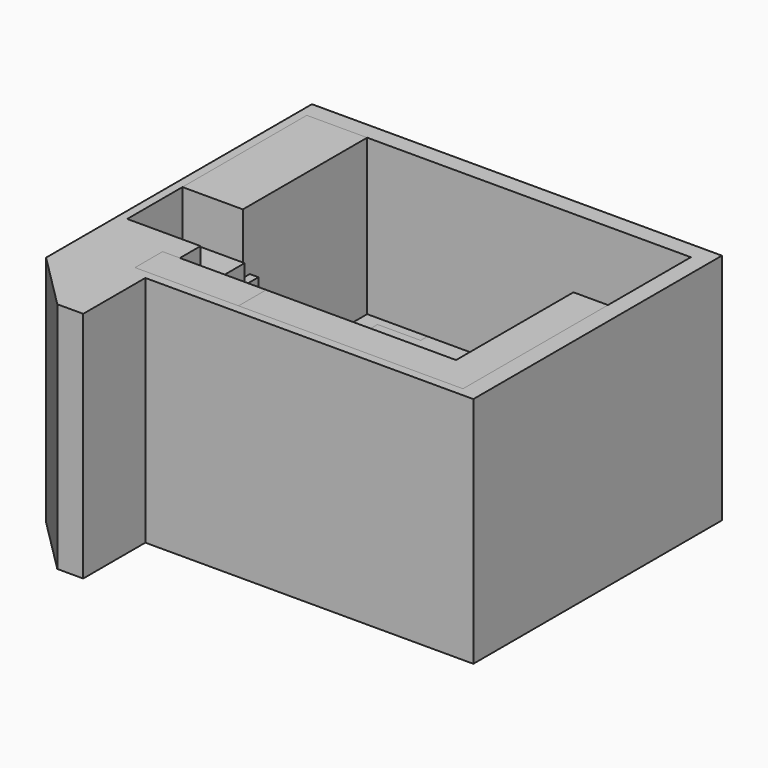
from build123d import *

# Parameters (mm, degrees)
F1_DEPTH       = 2700
F2_W           = 700
F2_H           = 2700
F3_DEPTH       = 1800
F4_W           = 500
F4_H           = 400
F5_DEPTH       = 750
F6_W           = 600
F6_H           = 900
F7_DEPTH       = 1200
F9_DEPTH       = 2100
F11_DEPTH      = 2000
F11_DEPTH_BACK = 200
F13_DEPTH      = 1200
F14_W          = 3850
F14_H          = 600
F15_DEPTH      = 900
F14_W_2        = 800
F14_H_2        = 900
F16_DEPTH      = 2000
F17_W          = 400
F17_H          = 400
F17_W_2        = 900
F17_W_3        = 500
F17_H_2        = 700
F17_H_3        = 100
F17_H_4        = 500
F18_DEPTH      = 2225
F17_H_5        = 300
F17_W_4        = 800
F17_H_6        = 1000
F17_W_5        = 450
F19_DEPTH      = 900
F17_W_6        = 300
F17_H_7        = 200


with BuildPart() as f1:
    # F0 (on Top) → F1 (new body)
    with BuildSketch(Plane.XY):
        Polygon((-1375, -2658.0309391022), (-1375, -1758.0309391022), (2425, -1758.0309391022), (2425, 1841.9690608978), (-2325, 1841.9690608978), (-2325, -2008.0309391022), (-1675, -2658.0309391022), align=None)
        Polygon((-2225, -958.0309391022), (-2225, 1641.9690608978), (2225, 1641.9690608978), (2225, -1658.0309391022), (-1375, -1658.0309391022), (-1375, -958.0309391022), align=None, mode=Mode.SUBTRACT)
    extrude(amount=F1_DEPTH)


with BuildPart() as f3:
    # F2 (on face) → F3 (new body)
    with BuildSketch(Plane.XZ.offset(-1641.9690608978)):
        with Locations((-1875, 1350)):
            Rectangle(F2_W, F2_H)
    extrude(amount=F3_DEPTH)


with BuildPart() as f5:
    # F4 (on Top) → F5 (new body)
    with BuildSketch(Plane.XY):
        with Locations((-325, -50)):
            Rectangle(F4_W, F4_H)
        Polygon((825, 300), (-75, 300), (-75, 150), (-75, -250), (-75, -400), (825, -400), (825, -250), (825, 150), align=None)
        with Locations((1075, -50)):
            Rectangle(F4_W, F4_H)
        Polygon((825, -400), (-75, -400), (-75, -550), (-75, -950), (-75, -1100), (825, -1100), (825, -950), (825, -550), align=None)
        with Locations((-325, -750)):
            Rectangle(F4_W, F4_H)
        with Locations((1075, -750)):
            Rectangle(F4_W, F4_H)
    extrude(amount=F5_DEPTH)


with BuildPart() as f7:
    # F6 (on face) → F7 (new body)
    with BuildSketch(Plane.XZ.offset(-1641.9690608978)):
        with Locations((1925, 450)):
            Rectangle(F6_W, F6_H)
    extrude(amount=F7_DEPTH)


with BuildPart() as f9:
    # F8 (on face) → F9 (new body, through all)
    with BuildSketch(Plane.XZ.offset(-441.9690608978)):
        Polygon((2215, 900), (2225, 900), (2225, 2700), (1825, 2700), (1825, 1500), (2215, 1500), align=None)
        Polygon((1625, 0), (2225, 0), (2225, 900), (2215, 900), (1625, 900), align=None)
    extrude(amount=F9_DEPTH)

    # F10 (on face) → F11 (join, two sides)
    with BuildSketch(Plane(origin=(1625, 0, 0), x_dir=(0, -1, 0), z_dir=(-1, 0, 0))) as f11_sk:
        Polygon((1648.0309391022, 900), (1658.0309391022, 900), (1658.0309391022, 2700), (1258.0309391022, 2700), (1258.0309391022, 1500), (1648.0309391022, 1500), align=None)
        Polygon((1258.0309391022, 0), (1658.0309391022, 0), (1658.0309391022, 900), (1648.0309391022, 900), (1258.0309391022, 900), align=None)
    extrude(amount=F11_DEPTH)
    extrude(f11_sk.sketch, amount=-F11_DEPTH_BACK)


with BuildPart() as f13:
    # F12 (on face) → F13 (new body)
    with BuildSketch(Plane(origin=(-375, 0, 0), x_dir=(0, -1, 0), z_dir=(-1, 0, 0))):
        Polygon((1658.0309391022, 0), (1658.0309391022, 2700), (1258.0309391022, 2700), (1258.0309391022, 1500), (1648.0309391022, 1500), (1648.0309391022, 900), (1258.0309391022, 900), (1258.0309391022, 0), align=None)
    extrude(amount=F13_DEPTH)


with BuildPart() as f15:
    # F14 (on Top) → F15 (new body)
    with BuildSketch(Plane.XY):
        with Locations((-300, 1341.9690608978)):
            Rectangle(F14_W, F14_H)
    extrude(amount=F15_DEPTH)


with BuildPart() as f16:
    # F14 (on Top) → F16 (new body)
    with BuildSketch(Plane.XY):
        with Locations((-1825, -508.0309391022)):
            Rectangle(F14_W_2, F14_H_2)
    extrude(amount=F16_DEPTH)


with BuildPart() as f18:
    # F17 (on Top) → F18 (new body)
    with BuildSketch(Plane.XY):
        with Locations((-75, -1458.0309391022)):
            Rectangle(F17_W, F17_H)
        with Locations((575, -1458.0309391022)):
            Rectangle(F17_W_2, F17_H)
        with Locations((1275, -1458.0309391022)):
            Rectangle(F17_W_3, F17_H)
        Polygon((1725, -1058.0309391022), (1525, -1258.0309391022), (1525, -1658.0309391022), (2225, -1658.0309391022), (2225, -1058.0309391022), align=None)
        Polygon((1825, -958.0309391022), (1725, -1058.0309391022), (2225, -1058.0309391022), (2225, -958.0309391022), align=None)
        with Locations((2025, -608.0309391022)):
            Rectangle(F17_W, F17_H_2)
        with Locations((2025, -208.0309391022)):
            Rectangle(F17_W, F17_H_3)
        with Locations((2025, 91.9690608978)):
            Rectangle(F17_W, F17_H_4)
    extrude(amount=F18_DEPTH)


with BuildPart() as f18b:
    # F17 (on Top) → F18, piece 2 (new body)
    with BuildSketch(Plane.XY):
        with Locations((2025, 791.9690608978)):
            Rectangle(F17_W, F17_H_5)
    extrude(amount=F18_DEPTH)


with BuildPart() as f18c:
    # F17 (on Top) → F18, piece 3 (new body)
    with BuildSketch(Plane.XY):
        with Locations((2025, 1391.9690608978)):
            Rectangle(F17_W, F17_H_3)
    extrude(amount=F18_DEPTH)


with BuildPart() as f18d:
    # F17 (on Top) → F18, piece 4 (new body)
    with BuildSketch(Plane.XY):
        with Locations((-1825, -608.0309391022)):
            Rectangle(F17_W_4, F17_H_2)
    extrude(amount=F18_DEPTH)


with BuildPart() as f18e:
    # F17 (on Top) → F18, piece 5 (new body)
    with BuildSketch(Plane.XY):
        with Locations((-2025, 1141.9690608978)):
            Rectangle(F17_W, F17_H_6)
    extrude(amount=F18_DEPTH)


with BuildPart() as f19:
    # F17 (on Top) → F19 (new body)
    with BuildSketch(Plane.XY):
        with Locations((-1075, 1291.9690608978)):
            Rectangle(F17_W_3, F17_H_4)
        with Locations((-600, 1591.9690608978)):
            Rectangle(F17_W_5, F17_H_3)
        with Locations((-150, 1591.9690608978)):
            Rectangle(F17_W_5, F17_H_3)
        with Locations((-150, 1291.9690608978)):
            Rectangle(F17_W_5, F17_H_4)
        with Locations((325, 1291.9690608978)):
            Rectangle(F17_W_3, F17_H_4)
        with Locations((-600, 1291.9690608978)):
            Rectangle(F17_W_5, F17_H_4)
        with Locations((-1075, 591.9690608978)):
            Rectangle(F17_W_3, F17_H_4)
        with Locations((-600, 591.9690608978)):
            Rectangle(F17_W_5, F17_H_4)
        with Locations((-600, 291.9690608978)):
            Rectangle(F17_W_5, F17_H_3)
        with Locations((-150, 991.9690608978)):
            Rectangle(F17_W_5, F17_H_3)
        with Locations((-600, 891.9690608978)):
            Rectangle(F17_W_5, F17_H_3)
        with Locations((-600, 991.9690608978)):
            Rectangle(F17_W_5, F17_H_3)
        with Locations((-150, 891.9690608978)):
            Rectangle(F17_W_5, F17_H_3)
        with Locations((-150, 591.9690608978)):
            Rectangle(F17_W_5, F17_H_4)
        with Locations((325, 591.9690608978)):
            Rectangle(F17_W_3, F17_H_4)
        with Locations((-150, 291.9690608978)):
            Rectangle(F17_W_5, F17_H_3)
    extrude(amount=F19_DEPTH)


with BuildPart() as f19b:
    # F17 (on Top) → F19, piece 2 (new body)
    with BuildSketch(Plane.XY):
        Polygon((1525, 1641.9690608978), (1525, 1441.9690608978), (1825, 1441.9690608978), (2225, 1441.9690608978), (2225, 1641.9690608978), align=None)
        with Locations((1675, 1391.9690608978)):
            Rectangle(F17_W_6, F17_H_3)
        with Locations((1675, 1141.9690608978)):
            Rectangle(F17_W_6, F17_H)
    extrude(amount=F19_DEPTH)


with BuildPart() as f19c:
    # F17 (on Top) → F19, piece 3 (new body)
    with BuildSketch(Plane.XY):
        Polygon((1525, -258.0309391022), (1525, -1058.0309391022), (1725, -1058.0309391022), (1825, -958.0309391022), (1825, -258.0309391022), align=None)
        Polygon((1525, -1058.0309391022), (1025, -1058.0309391022), (1025, -1258.0309391022), (1525, -1258.0309391022), (1725, -1058.0309391022), align=None)
        with Locations((575, -1158.0309391022)):
            Rectangle(F17_W_2, F17_H_7)
        with Locations((-75, -1158.0309391022)):
            Rectangle(F17_W, F17_H_7)
        Polygon((-275, -1258.0309391022), (-275, -1058.0309391022), (-475, -1258.0309391022), (-475, -1658.0309391022), (-275, -1658.0309391022), align=None)
    extrude(amount=F19_DEPTH)


solid = Compound([f1.part, f3.part, f5.part, f7.part, f9.part, f13.part, f15.part, f16.part, f18.part, f18b.part, f18c.part, f18d.part, f18e.part, f19.part, f19b.part, f19c.part])
